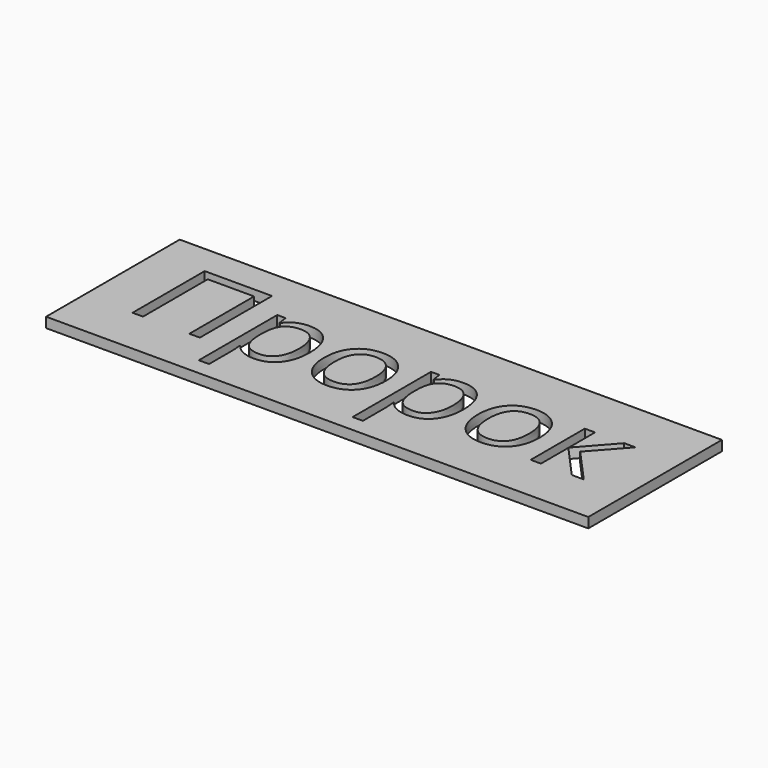
from build123d import *

# Parameters (mm, degrees)
F0_W         = 107.6828949153
F0_H         = 33.1712849438
F1_DEPTH     = 2
F2_TEXT_SIZE = 25.0985018081
F3_DEPTH     = 25


# Not quite as in the source:
# - Text() gives the source's letters only with a copy of the font that has no kerning and outlines rounded to 1/6400 em; it was checked with that copy


with BuildPart() as f1:
    # F0 (on Top) → F1 (new body)
    with BuildSketch(Plane.XY):
        with Locations((8.4205474705, 28.5879541188)):
            Rectangle(F0_W, F0_H)
    extrude(amount=F1_DEPTH)

    # F2 (on face) → F3 (cut)
    with BuildSketch(Plane.XY.offset(2)):
        with Locations((-38.2420420647, 21.4090943336)):
            Text('Пророк', F2_TEXT_SIZE, font='Open Sans', text_align=(TextAlign.LEFT, TextAlign.BOTTOM))
    extrude(amount=-F3_DEPTH, mode=Mode.SUBTRACT)


solid = f1.part
